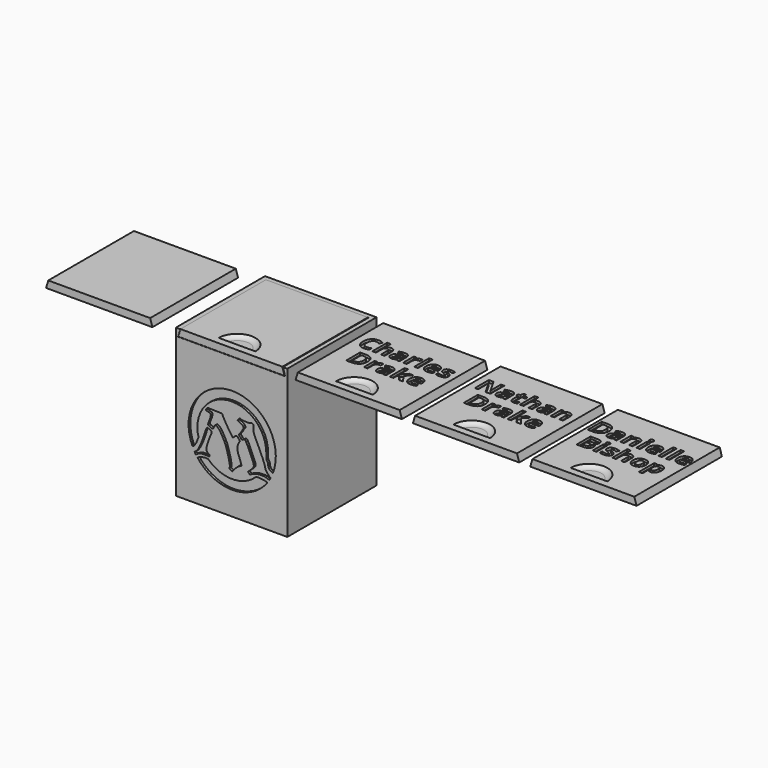
from build123d import *

# Parameters (mm, degrees)
F0_W          = 76
F0_H          = 76
F0_W_2        = 70
F0_H_2        = 70
F1_DEPTH      = 101
F2_T          = -3
F4_DEPTH      = 1.5
F6_DEPTH      = 1.5
F8_DEPTH      = 73
F10_DEPTH     = 73
F13_DEPTH     = 2
F14_T2_ANGLE  = 180
F15_DEPTH     = 0.2
F17_TEXT_SIZE = 16.6666666667
F18_DEPTH     = 1.7
F20_TEXT_SIZE = 16.6666666667
F21_DEPTH     = 1.7
F23_TEXT_SIZE = 16.6666666667
F24_DEPTH     = 1.7


# Not quite as in the source:
# - a fillet or chamfer that OpenCascade refuses, or shapes differently, is made with other operations: its cross-section is extruded or revolved along the edge and cut away or added
# - ends of sketch curves that miss each other by under 0.0002 mm in the source are joined
# - Text() gives the source's letters only with a copy of the font that has no kerning and outlines rounded to 1/6400 em; it was checked with that copy


with BuildPart() as f1:
    # F0 (on Top) → F1 (new body)
    with BuildSketch(Plane.XY):
        Rectangle(F0_W, F0_H)
        Rectangle(F0_W_2, F0_H_2, mode=Mode.SUBTRACT)
        Rectangle(F0_W_2, F0_H_2)
    extrude(amount=F1_DEPTH)

    # F2
    f2_openings = [f1.faces().sort_by_distance(p)[0] for p in [
        (0, 0, 101),
    ]]
    offset(amount=F2_T, openings=f2_openings)

    # F3 (on face) → F4 (cut)
    with BuildSketch(Plane.XZ.offset(38)):
        Polygon((-0.4040717683, 75.5102922818), (-4.3064167683, 75.1443172818), (-8.1267827683, 74.2684942818), (-11.7988487683, 72.8980352818), (-15.2588887683, 71.0567302818), (-18.4468317683, 68.7765432818), (-21.3073387683, 66.0970412818), (-23.7907747683, 63.0647482818), (-25.8540087683, 59.7322922818), (-27.4612537683, 56.1575202818), (-28.5845947683, 52.4024732818), (-29.2045377683, 48.5323482818), (-29.3103197683, 44.6143062818), (-28.9001077683, 40.7163642818), (-27.9810187683, 36.9061802818), (-26.6491757683, 33.4574742818), (-26.3627217683, 33.5535842818), (-26.1486297683, 33.6569762818), (-25.9661717683, 33.7809942818), (-25.2596027683, 34.5743172818), (-24.0698427683, 36.3678992818), (-22.4587547683, 40.3571682818), (-23.0023267683, 42.0458712818), (-23.3073607683, 43.9042412818), (-23.3334187683, 45.7713752818), (-23.3314467683, 46.0294862818), (-23.3266527683, 46.2869182818), (-23.3085647683, 46.8008852818), (-23.2385757683, 47.8249932818), (-23.0833227683, 49.1302592818), (-22.3553197683, 52.4062522818), (-21.1616097683, 55.5485932818), (-19.5282317683, 58.4865122818), (-17.4891687683, 61.1588742818), (-15.0868497683, 63.5100752818), (-12.3712617683, 65.4912032818), (-9.3989017683, 67.0610272818), (-6.2316137683, 68.1868982818), (-2.9439647683, 68.8436392818), (-2.8517567683, 68.8550622818), (-2.7680227683, 68.8651182818), (-2.6006807683, 68.8843102818), (-2.2602087683, 68.9196172818), (0.4207302317, 69.0225062818), (3.7255052317, 68.7861422818), (6.9670582317, 68.0809872818), (10.0752632317, 66.9216932818), (12.9868392317, 65.3318452818), (15.6425272317, 63.3438232818), (17.9882562317, 60.9980982818), (19.9762742317, 58.3424102818), (21.5661222317, 55.4308302818), (22.7254202317, 52.3226262818), (23.4287152317, 49.0896022818), (23.4416052317, 48.9988102818), (23.4530092317, 48.9163652818), (23.4749022317, 48.7515842818), (23.5158092317, 48.4162602818), (23.6666292317, 45.7787222818), (23.6513842317, 42.5201402818), (23.6885372317, 42.1498222818), (23.7861742317, 41.8070362818), (24.1682732317, 41.1271972818), (24.6231682317, 40.4245682818), (24.7742252317, 40.0015192818), (24.8532512317, 39.5750872818), (25.0745872317, 37.9653192818), (25.3304182317, 37.2385912818), (25.5115312317, 36.9209862818), (25.7367912317, 36.6349522818), (26.3194922317, 36.1164552818), (26.9907082317, 35.6731752818), (28.1405202317, 35.0311852818), (29.2599612317, 38.4858372818), (29.9675152317, 42.3409122818), (30.1621242317, 46.2555522818), (29.8404132317, 50.1617952818), (29.0079742317, 53.9918382818), (27.6792442317, 57.6792162818), (25.8772982317, 61.1599112818), (23.6334062317, 64.3734962818), (20.9865192317, 67.2642132818), (17.9825872317, 69.7818692818), (14.6737442317, 71.8827712818), (11.1174252317, 73.5304482818), (7.3753592317, 74.6963022818), (3.5125112317, 75.3600862818), align=None)
        Polygon((6.6751642317, 32.9071462818), (6.6608672317, 32.9569952818), (6.6454502317, 33.0107452818), (6.6146502317, 33.1180932818), (6.5538172317, 33.3295452818), (5.6720412317, 36.0862752818), (4.4881632317, 39.2291942818), (4.0456822317, 40.8744592818), (3.9273242317, 41.7380692818), (3.9263262317, 42.6140772818), (4.0560452317, 43.4793802818), (4.3012332317, 44.3147342818), (4.9789142317, 45.8947672818), (5.5673262317, 46.7298182818), (5.5872702317, 46.7855902818), (5.5946772317, 46.8564762818), (5.5749522317, 47.0902502818), (5.5417852317, 47.3312342818), (5.5148902317, 47.4229682818), (5.4906342317, 47.4574172818), (4.1636202317, 48.9975312818), (3.9991122317, 49.1464282818), (3.8212272317, 49.2624842818), (3.6371602317, 49.3319992818), (3.4438702317, 49.3514842818), (2.9793182317, 49.2897472818), (2.7750402317, 49.2257002818), (2.5926592317, 49.1334292818), (0.8799152317, 47.6042772818), (0.2146652317, 48.4917962818), (-1.6956667683, 51.1786762818), (-3.4535407683, 53.9708882818), (-5.1146707683, 56.8205992818), (-6.5391337683, 59.6266332818), (-16.4574717683, 59.9183512818), (-17.3783847683, 58.6290542818), (-17.6114987683, 58.2852152818), (-17.5473197683, 58.2122772818), (-17.2430877683, 57.9413892818), (-17.1002837683, 57.8581352818), (-16.9522457683, 57.8031692818), (-16.1054727683, 57.6989872818), (-15.2653657683, 57.4011922818), (-14.8346957683, 57.1973742818), (-14.6073227683, 57.0759572818), (-14.3969047683, 56.9171192818), (-14.2963787683, 56.7989642818), (-14.2235407683, 56.6640842818), (-14.1829787683, 56.5193962818), (-14.1671697683, 56.3697062818), (-14.2065517683, 55.8781422818), (-14.5779357683, 54.1757612818), (-15.2036547683, 52.5433812818), (-15.8162127683, 50.9462142818), (-15.9550077683, 50.5445352818), (-16.0361087683, 50.1631322818), (-16.0298377683, 50.0151142818), (-15.9856117683, 49.8680142818), (-15.9031267683, 49.7260382818), (-15.7900397683, 49.6017142818), (-15.6523917683, 49.5030882818), (-15.4873997683, 49.4226182818), (-15.0883547683, 49.2697922818), (-14.2998287683, 48.9139002818), (-13.5130627683, 48.5047732818), (-13.3405107683, 48.4386472818), (-13.1764937683, 48.4053592818), (-13.1134217683, 48.4038392818), (-13.0535567683, 48.4109422818), (-12.9014757683, 48.4612962818), (-12.7527247683, 48.5495352818), (-12.6178257683, 48.6648692818), (-12.3813457683, 48.9753872818), (-12.0048267683, 49.7100382818), (-11.6465307683, 50.5380912818), (-11.5449677683, 50.7636942818), (-11.4653817683, 50.8848622818), (-11.3646547683, 50.9928432818), (-11.2350897683, 51.0807082818), (-11.0845497683, 51.1331702818), (-10.9318587683, 51.1503912818), (-10.7798917683, 51.1432752818), (-10.5186387683, 51.0872102818), (-10.2778097683, 50.9907612818), (-9.8805267683, 50.7485262818), (-9.1811767683, 50.1877902818), (-7.9924437683, 48.8806012818), (-6.2182927683, 45.8939282818), (-4.9789597683, 43.5191462818), (-3.8746507683, 41.0665042818), (-2.3727067683, 35.9256042818), (-1.7384157683, 33.3403722818), (-1.2292867683, 30.6815502818), (-1.1727277683, 29.9759482818), (-1.2474887683, 29.2811342818), (-1.4100077683, 28.6041812818), (-1.4760157683, 28.4177382818), (-1.5646707683, 28.2511322818), (-1.5909377683, 28.2048122818), (-1.4712677683, 28.1729212818), (-1.1100707683, 28.0248972818), (-0.5449877683, 27.6707032818), (0.0221042317, 27.3344842818), (0.3247722317, 27.1199452818), (0.4369792317, 26.9996132818), (0.5893612317, 27.3901922818), (0.8999862317, 27.8839222818), (1.6747112317, 28.6821742818), (3.1945492317, 30.2222592818), (3.9915072317, 30.9908082818), (4.9131732317, 31.5827902818), (5.8692902317, 32.1576632818), (6.1356392317, 32.2904342818), (6.4263152317, 32.3874972818), (6.7308582317, 32.4260882818), (6.7661262317, 32.4256062818), (6.7659022317, 32.5469872818), align=None)
        Polygon((19.4331262317, 45.6693772818), (18.7905172317, 47.0654182818), (16.2318482317, 52.3506892818), (15.1644112317, 55.0983982818), (14.9473782317, 55.8312792818), (14.8689412317, 56.6017252818), (14.9362672317, 58.0945852818), (15.0656712317, 59.5406802818), (15.0657572317, 59.7102412818), (15.0465212317, 59.8561612818), (15.0290602317, 59.9060242818), (14.9943362317, 59.9406242818), (14.9481502317, 59.9726752818), (14.3079202317, 60.3253332818), (14.0012052317, 60.5074992818), (13.9527942317, 60.5289102818), (13.9119982317, 60.5386352818), (13.8657752317, 60.5407872818), (13.8229512317, 60.5363292818), (13.1155542317, 60.2902882818), (11.6562662317, 60.0146172818), (10.1606882317, 59.9238292818), (8.6832032317, 60.0608922818), (7.1986622317, 60.1859402818), (5.7808482317, 60.6009662818), (5.6320202317, 60.6314572818), (5.5014052317, 60.6331252818), (5.4675822317, 60.6252572818), (5.4331542317, 60.6097732818), (5.3273292317, 60.5312812818), (4.8500532317, 59.9977642818), (4.3934102317, 59.4557892818), (4.2193062317, 59.1814072818), (4.1707162317, 59.0522822818), (4.1465932317, 58.9122982818), (4.1488822317, 58.8632422818), (4.1756692317, 58.8402332818), (4.3037862317, 58.7754472818), (4.4883272317, 58.7116562818), (5.2434032317, 58.4221502818), (6.5230432317, 57.7417082818), (7.1513012317, 57.3604402818), (7.4752972317, 57.1388062818), (7.7765062317, 56.8636292818), (8.0220052317, 56.5262402818), (8.1952242317, 56.1418132818), (8.2518352317, 55.9184262818), (8.2693342317, 55.6885632818), (8.2346242317, 55.4615802818), (8.1506472317, 55.2412382818), (7.2537562317, 54.0066212818), (6.5438492317, 52.7462712818), (6.1004322317, 52.1138612818), (5.5254822317, 51.5674102818), (5.2518382317, 51.3216692818), (5.1587992317, 51.2121672818), (5.0934362317, 51.1030722818), (5.0563012317, 50.9904402818), (5.0456822317, 50.8624742818), (5.0619862317, 50.7251232818), (5.1023522317, 50.5949512818), (5.2591022317, 50.3069972818), (5.4589892317, 50.0274912818), (5.9121182317, 49.4785182818), (6.4025522317, 48.9393162818), (6.6525292317, 48.6829932818), (6.7698002317, 48.5869832818), (6.8877992317, 48.5156942818), (7.0169432317, 48.4675752818), (7.1683632317, 48.4341952818), (7.5121262317, 48.3911902818), (7.5647132317, 48.3935052818), (7.6128132317, 48.4023992818), (7.6542592317, 48.4180422818), (7.6940762317, 48.4412912818), (7.9739342317, 48.6789562818), (8.3147012317, 48.9021112818), (8.5317432317, 48.9879102818), (8.6601542317, 49.0161072818), (8.7927192317, 49.0248262818), (8.9276212317, 49.0086632818), (9.0615762317, 48.9674112818), (9.2705782317, 48.8508882818), (9.4471912317, 48.6982772818), (9.5963252317, 48.5211472818), (10.9501062317, 45.8788312818), (14.8118052317, 36.9356832818), (15.1745822317, 35.7297962818), (15.2007112317, 35.3804292818), (15.1718342317, 35.0381422818), (15.0947432317, 34.7059992818), (14.9739262317, 34.3865492818), (14.6478182317, 33.8273462818), (14.2412732317, 33.3228582818), (13.3561822317, 32.4385592818), (11.5900882317, 30.8298382818), (11.3804882317, 30.6068212818), (11.2804402317, 30.4923272818), (11.2343352317, 30.4290342818), (11.4540852317, 30.2101272818), (11.9326672317, 29.7310812818), (12.2636792317, 29.2794712818), (12.5302522317, 29.0761602818), (13.6507782317, 29.7814472818), (15.0438642317, 30.3694292818), (16.4672942317, 30.8459912818), (17.9437402317, 31.1700302818), (19.9820472317, 31.3222472818), (22.0387242317, 31.3013952818), (24.0452282317, 30.8220302818), (25.7646972317, 30.2022802818), (26.0578182317, 30.6861072818), (26.4382662317, 31.3522482818), (26.6824652317, 31.8066462818), (26.1440332317, 32.0837282818), (25.4514272317, 32.6360592818), (24.3573592317, 33.9509892818), (23.3797372317, 35.3647242818), (23.0557862317, 36.1783372818), (22.8748422317, 37.0074102818), (22.2124702317, 39.0857212818), (21.2855852317, 41.4764132818), align=None)
        Polygon((24.4773142317, 28.3088662818), (23.8207522317, 28.5389362818), (22.8023862317, 28.7482302818), (20.6941912317, 29.0297302818), (18.5800212317, 29.3093132818), (17.5534582317, 29.2993892818), (16.6022162317, 29.0879432818), (14.1644562317, 27.0214872818), (11.3933272317, 25.2757592818), (8.4043872317, 23.9367142818), (5.2569512317, 23.0309612818), (2.0134682317, 22.5764432818), (-1.2616947683, 22.5821942818), (-4.5035707683, 23.0480862818), (-7.6478027683, 23.9648982818), (-10.6320197683, 25.3144162818), (-13.3970037683, 27.0698672818), (-15.8302047683, 29.1471782818), (-16.7546557683, 29.3824352818), (-17.7254377683, 29.4338512818), (-19.7580277683, 29.1214912818), (-21.7231527683, 28.5883942818), (-22.5988087683, 28.1437902818), (-23.2128767683, 27.7230022818), (-20.9627687683, 25.0850702818), (-18.2065577683, 22.5727732818), (-15.1576687683, 20.4250672818), (-11.8640407683, 18.6756872818), (-8.3774187683, 17.3521212818), (-4.7525907683, 16.4751892818), (-1.0465357683, 16.0586582818), (2.6825072317, 16.1090752818), (6.3759462317, 16.6256492818), (9.9757372317, 17.6002622818), (13.4253012317, 19.0175982818), (16.6704352317, 20.8553832818), (19.6601432317, 23.0847432818), (22.3474262317, 25.6706302818), align=None)
        Polygon((-25.0980437683, 30.8046492818), (-25.2241227683, 30.7627782818), (-25.2725437683, 30.7408502818), (-24.8979357683, 29.7951742818), (-24.4477487683, 29.1557772818), (-24.1651227683, 29.4026772818), (-23.7359097683, 29.6720222818), (-22.8871427683, 30.1942022818), (-21.0300087683, 30.8732472818), (-20.0450237683, 31.0837882818), (-19.0547127683, 31.1374072818), (-17.0978867683, 31.1274692818), (-14.9320787683, 30.9441102818), (-14.9283877683, 31.6998682818), (-14.9593187683, 31.9267422818), (-14.9844177683, 32.0097652818), (-15.0212367683, 32.0800272818), (-15.0751587683, 32.1458972818), (-15.1449537683, 32.2080712818), (-15.3449557683, 32.3361442818), (-16.2849107683, 32.8504562818), (-16.6852527683, 33.2939272818), (-16.9767747683, 33.8013592818), (-17.1642547683, 34.3475072818), (-17.2369137683, 34.9231002818), (-17.0860877683, 36.0103432818), (-16.4812087683, 38.0341712818), (-15.1390857683, 42.0066832818), (-13.5565947683, 45.8275382818), (-13.5383627683, 46.2129562818), (-13.5691997683, 46.3795032818), (-13.5909727683, 46.4294732818), (-13.6209857683, 46.4718842818), (-13.7531897683, 46.5867042818), (-13.9315137683, 46.7011812818), (-14.3148647683, 46.9373762818), (-14.4489887683, 47.0177382818), (-14.5819327683, 47.0952882818), (-14.8495357683, 47.2429052818), (-15.4132607683, 47.5133822818), (-15.8733647683, 47.7120992818), (-16.2711577683, 47.8688382818), (-16.3399887683, 47.8798172818), (-16.4219987683, 47.8816622818), (-16.5053437683, 47.8724262818), (-16.5866377683, 47.8524302818), (-16.6620077683, 47.8226722818), (-16.7225117683, 47.7879752818), (-16.8481937683, 47.6751812818), (-17.0781837683, 47.3335572818), (-17.7951467683, 45.6839642818), (-19.1565487683, 41.4368052818), (-20.7460367683, 37.2350202818), (-21.5742747683, 35.3318482818), (-22.5395037683, 33.4935902818), (-23.7372817683, 31.7584062818), (-24.5687447683, 31.0810082818), (-24.8143747683, 30.9182372818), align=None)
    extrude(amount=-F4_DEPTH, mode=Mode.SUBTRACT)

    # F5 (on face) → F6 (cut)
    with BuildSketch(Plane(origin=(0, 38, 0), x_dir=(-1, 0, 0), z_dir=(0, 1, 0))):
        Polygon((0.0653751924, 80.0444194725), (-3.8369698076, 79.6784444725), (-7.6573358076, 78.8026214725), (-11.3294018076, 77.4321624725), (-14.7894418076, 75.5908574725), (-17.9773848076, 73.3106704725), (-20.8378918076, 70.6311684725), (-23.3213278076, 67.5988754725), (-25.3845618076, 64.2664194725), (-26.9918068076, 60.6916474725), (-28.1151478076, 56.9366004725), (-28.7350908076, 53.0664754725), (-28.8408728076, 49.1484334725), (-28.4306608076, 45.2504914725), (-27.5115718076, 41.4403074725), (-26.1797288076, 37.9916014725), (-25.8932748076, 38.0877114725), (-25.6791828076, 38.1911034725), (-25.4967248076, 38.3151214725), (-24.7901558076, 39.1084444725), (-23.6003958076, 40.9020264725), (-21.9893078076, 44.8912954725), (-22.5328798076, 46.5799984725), (-22.8379138076, 48.4383684725), (-22.8639718076, 50.3055024725), (-22.8619998076, 50.5636134725), (-22.8572058076, 50.8210454725), (-22.8391178076, 51.3350124725), (-22.7691288076, 52.3591204725), (-22.6138758076, 53.6643864725), (-21.8858728076, 56.9403794725), (-20.6921628076, 60.0827204725), (-19.0587848076, 63.0206394725), (-17.0197218076, 65.6930014725), (-14.6174028076, 68.0442024725), (-11.9018148076, 70.0253304725), (-8.9294548076, 71.5951544725), (-5.7621668076, 72.7210254725), (-2.4745178076, 73.3777664725), (-2.3823098076, 73.3891894725), (-2.2985758076, 73.3992454725), (-2.1312338076, 73.4184374725), (-1.7907618076, 73.4537444725), (0.8901771924, 73.5566334725), (4.1949521924, 73.3202694725), (7.4365051924, 72.6151144725), (10.5447101924, 71.4558204725), (13.4562861924, 69.8659724725), (16.1119741924, 67.8779504725), (18.4577031924, 65.5322254725), (20.4457211924, 62.8765374725), (22.0355691924, 59.9649574725), (23.1948671924, 56.8567534725), (23.8981621924, 53.6237294725), (23.9110521924, 53.5329374725), (23.9224561924, 53.4504924725), (23.9443491924, 53.2857114725), (23.9852561924, 52.9503874725), (24.1360761924, 50.3128494725), (24.1208311924, 47.0542674725), (24.1579841924, 46.6839494725), (24.2556211924, 46.3411634725), (24.6377201924, 45.6613244725), (25.0926151924, 44.9586954725), (25.2436721924, 44.5356464725), (25.3226981924, 44.1092144725), (25.5440341924, 42.4994464725), (25.7998651924, 41.7727184725), (25.9809781924, 41.4551134725), (26.2062381924, 41.1690794725), (26.7889391924, 40.6505824725), (27.4601551924, 40.2073024725), (28.6099671924, 39.5653124725), (29.7294081924, 43.0199644725), (30.4369621924, 46.8750394725), (30.6315711924, 50.7896794725), (30.3098601924, 54.6959224725), (29.4774211924, 58.5259654725), (28.1486911924, 62.2133434725), (26.3467451924, 65.6940384725), (24.1028531924, 68.9076234725), (21.4559661924, 71.7983404725), (18.4520341924, 74.3159964725), (15.1431911924, 76.4168984725), (11.5868721924, 78.0645754725), (7.8448061924, 79.2304294725), (3.9819581924, 79.8942134725), align=None)
        Polygon((7.1446111924, 37.4412734725), (7.1303141924, 37.4911224725), (7.1148971924, 37.5448724725), (7.0840971924, 37.6522204725), (7.0232641924, 37.8636724725), (6.1414881924, 40.6204024725), (4.9576101924, 43.7633214725), (4.5151291924, 45.4085864725), (4.3967711924, 46.2721964725), (4.3957731924, 47.1482044725), (4.5254921924, 48.0135074725), (4.7706801924, 48.8488614725), (5.4483611924, 50.4288944725), (6.0367731924, 51.2639454725), (6.0567171924, 51.3197174725), (6.0641241924, 51.3906034725), (6.0443991924, 51.6243774725), (6.0112321924, 51.8653614725), (5.9843371924, 51.9570954725), (5.9600811924, 51.9915444725), (4.6330671924, 53.5316584725), (4.4685591924, 53.6805554725), (4.2906741924, 53.7966114725), (4.1066071924, 53.8661264725), (3.9133171924, 53.8856114725), (3.4487651924, 53.8238744725), (3.2444871924, 53.7598274725), (3.0621061924, 53.6675564725), (1.3493621924, 52.1384044725), (0.6841121924, 53.0259234725), (-1.2262198076, 55.7128034725), (-2.9840938076, 58.5050154725), (-4.6452238076, 61.3547264725), (-6.0696868076, 64.1607604725), (-15.9880248076, 64.4524784725), (-16.9089378076, 63.1631814725), (-17.1420518076, 62.8193424725), (-17.0778728076, 62.7464044725), (-16.7736408076, 62.4755164725), (-16.6308368076, 62.3922624725), (-16.4827988076, 62.3372964725), (-15.6360258076, 62.2331144725), (-14.7959188076, 61.9353194725), (-14.3652488076, 61.7315014725), (-14.1378758076, 61.6100844725), (-13.9274578076, 61.4512464725), (-13.8269318076, 61.3330914725), (-13.7540938076, 61.1982114725), (-13.7135318076, 61.0535234725), (-13.6977228076, 60.9038334725), (-13.7371048076, 60.4122694725), (-14.1084888076, 58.7098884725), (-14.7342078076, 57.0775084725), (-15.3467658076, 55.4803414725), (-15.4855608076, 55.0786624725), (-15.5666618076, 54.6972594725), (-15.5603908076, 54.5492414725), (-15.5161648076, 54.4021414725), (-15.4336798076, 54.2601654725), (-15.3205928076, 54.1358414725), (-15.1829448076, 54.0372154725), (-15.0179528076, 53.9567454725), (-14.6189078076, 53.8039194725), (-13.8303818076, 53.4480274725), (-13.0436158076, 53.0389004725), (-12.8710638076, 52.9727744725), (-12.7070468076, 52.9394864725), (-12.6439748076, 52.9379664725), (-12.5841098076, 52.9450694725), (-12.4320288076, 52.9954234725), (-12.2832778076, 53.0836624725), (-12.1483788076, 53.1989964725), (-11.9118988076, 53.5095144725), (-11.5353798076, 54.2441654725), (-11.1770838076, 55.0722184725), (-11.0755208076, 55.2978214725), (-10.9959348076, 55.4189894725), (-10.8952078076, 55.5269704725), (-10.7656428076, 55.6148354725), (-10.6151028076, 55.6672974725), (-10.4624118076, 55.6845184725), (-10.3104448076, 55.6774024725), (-10.0491918076, 55.6213374725), (-9.8083628076, 55.5248884725), (-9.4110798076, 55.2826534725), (-8.7117298076, 54.7219174725), (-7.5229968076, 53.4147284725), (-5.7488458076, 50.4280554725), (-4.5095128076, 48.0532734725), (-3.4052038076, 45.6006314725), (-1.9032598076, 40.4597314725), (-1.2689688076, 37.8744994725), (-0.7598398076, 35.2156774725), (-0.7032808076, 34.5100754725), (-0.7780418076, 33.8152614725), (-0.9405608076, 33.1383084725), (-1.0065688076, 32.9518654725), (-1.0952238076, 32.7852594725), (-1.1214908076, 32.7389394725), (-1.0018208076, 32.7070484725), (-0.6406238076, 32.5590244725), (-0.0755408076, 32.2048304725), (0.4915511924, 31.8686114725), (0.7942191924, 31.6540724725), (0.9064261924, 31.5337404725), (1.0588081924, 31.9243194725), (1.3694331924, 32.4180494725), (2.1441581924, 33.2163014725), (3.6639961924, 34.7563864725), (4.4609541924, 35.5249354725), (5.3826201924, 36.1169174725), (6.3387371924, 36.6917904725), (6.6050861924, 36.8245614725), (6.8957621924, 36.9216244725), (7.2003051924, 36.9602154725), (7.2355731924, 36.9597334725), (7.2353491924, 37.0811144725), align=None)
        Polygon((19.9025731924, 50.2035044725), (19.2599641924, 51.5995454725), (16.7012951924, 56.8848164725), (15.6338581924, 59.6325254725), (15.4168251924, 60.3654064725), (15.3383881924, 61.1358524725), (15.4057141924, 62.6287124725), (15.5351181924, 64.0748074725), (15.5352041924, 64.2443684725), (15.5159681924, 64.3902884725), (15.4985071924, 64.4401514725), (15.4637831924, 64.4747514725), (15.4175971924, 64.5068024725), (14.7773671924, 64.8594604725), (14.4706521924, 65.0416264725), (14.4222411924, 65.0630374725), (14.3814451924, 65.0727624725), (14.3352221924, 65.0749144725), (14.2923981924, 65.0704564725), (13.5850011924, 64.8244154725), (12.1257131924, 64.5487444725), (10.6301351924, 64.4579564725), (9.1526501924, 64.5950194725), (7.6681091924, 64.7200674725), (6.2502951924, 65.1350934725), (6.1014671924, 65.1655844725), (5.9708521924, 65.1672524725), (5.9370291924, 65.1593844725), (5.9026011924, 65.1439004725), (5.7967761924, 65.0654084725), (5.3195001924, 64.5318914725), (4.8628571924, 63.9899164725), (4.6887531924, 63.7155344725), (4.6401631924, 63.5864094725), (4.6160401924, 63.4464254725), (4.6183291924, 63.3973694725), (4.6451161924, 63.3743604725), (4.7732331924, 63.3095744725), (4.9577741924, 63.2457834725), (5.7128501924, 62.9562774725), (6.9924901924, 62.2758354725), (7.6207481924, 61.8945674725), (7.9447441924, 61.6729334725), (8.2459531924, 61.3977564725), (8.4914521924, 61.0603674725), (8.6646711924, 60.6759404725), (8.7212821924, 60.4525534725), (8.7387811924, 60.2226904725), (8.7040711924, 59.9957074725), (8.6200941924, 59.7753654725), (7.7232031924, 58.5407484725), (7.0132961924, 57.2803984725), (6.5698791924, 56.6479884725), (5.9949291924, 56.1015374725), (5.7212851924, 55.8557964725), (5.6282461924, 55.7462944725), (5.5628831924, 55.6371994725), (5.5257481924, 55.5245674725), (5.5151291924, 55.3966014725), (5.5314331924, 55.2592504725), (5.5717991924, 55.1290784725), (5.7285491924, 54.8411244725), (5.9284361924, 54.5616184725), (6.3815651924, 54.0126454725), (6.8719991924, 53.4734434725), (7.1219761924, 53.2171204725), (7.2392471924, 53.1211104725), (7.3572461924, 53.0498214725), (7.4863901924, 53.0017024725), (7.6378101924, 52.9683224725), (7.9815731924, 52.9253174725), (8.0341601924, 52.9276324725), (8.0822601924, 52.9365264725), (8.1237061924, 52.9521694725), (8.1635231924, 52.9754184725), (8.4433811924, 53.2130834725), (8.7841481924, 53.4362384725), (9.0011901924, 53.5220374725), (9.1296011924, 53.5502344725), (9.2621661924, 53.5589534725), (9.3970681924, 53.5427904725), (9.5310231924, 53.5015384725), (9.7400251924, 53.3850154725), (9.9166381924, 53.2324044725), (10.0657721924, 53.0552744725), (11.4195531924, 50.4129584725), (15.2812521924, 41.4698104725), (15.6440291924, 40.2639234725), (15.6701581924, 39.9145564725), (15.6412811924, 39.5722694725), (15.5641901924, 39.2401264725), (15.4433731924, 38.9206764725), (15.1172651924, 38.3614734725), (14.7107201924, 37.8569854725), (13.8256291924, 36.9726864725), (12.0595351924, 35.3639654725), (11.8499351924, 35.1409484725), (11.7498871924, 35.0264544725), (11.7037821924, 34.9631614725), (11.9235321924, 34.7442544725), (12.4021141924, 34.2652084725), (12.7331261924, 33.8135984725), (12.9996991924, 33.6102874725), (14.1202251924, 34.3155744725), (15.5133111924, 34.9035564725), (16.9367411924, 35.3801184725), (18.4131871924, 35.7041574725), (20.4514941924, 35.8563744725), (22.5081711924, 35.8355224725), (24.5146751924, 35.3561574725), (26.2341441924, 34.7364074725), (26.5272651924, 35.2202344725), (26.9077131924, 35.8863754725), (27.1519121924, 36.3407734725), (26.6134801924, 36.6178554725), (25.9208741924, 37.1701864725), (24.8268061924, 38.4851164725), (23.8491841924, 39.8988514725), (23.5252331924, 40.7124644725), (23.3442891924, 41.5415374725), (22.6819171924, 43.6198484725), (21.7550321924, 46.0105404725), align=None)
        Polygon((24.9467611924, 32.8429934725), (24.2901991924, 33.0730634725), (23.2718331924, 33.2823574725), (21.1636381924, 33.5638574725), (19.0494681924, 33.8434404725), (18.0229051924, 33.8335164725), (17.0716631924, 33.6220704725), (14.6339031924, 31.5556144725), (11.8627741924, 29.8098864725), (8.8738341924, 28.4708414725), (5.7263981924, 27.5650884725), (2.4829151924, 27.1105704725), (-0.7922478076, 27.1163214725), (-4.0341238076, 27.5822134725), (-7.1783558076, 28.4990254725), (-10.1625728076, 29.8485434725), (-12.9275568076, 31.6039944725), (-15.3607578076, 33.6813054725), (-16.2852088076, 33.9165624725), (-17.2559908076, 33.9679784725), (-19.2885808076, 33.6556184725), (-21.2537058076, 33.1225214725), (-22.1293618076, 32.6779174725), (-22.7434298076, 32.2571294725), (-20.4933218076, 29.6191974725), (-17.7371108076, 27.1069004725), (-14.6882218076, 24.9591944725), (-11.3945938076, 23.2098144725), (-7.9079718076, 21.8862484725), (-4.2831438076, 21.0093164725), (-0.5770888076, 20.5927854725), (3.1519541924, 20.6432024725), (6.8453931924, 21.1597764725), (10.4451841924, 22.1343894725), (13.8947481924, 23.5517254725), (17.1398821924, 25.3895104725), (20.1295901924, 27.6188704725), (22.8168731924, 30.2047574725), align=None)
        Polygon((-24.6285968076, 35.3387764725), (-24.7546758076, 35.2969054725), (-24.8030968076, 35.2749774725), (-24.4284888076, 34.3293014725), (-23.9783018076, 33.6899044725), (-23.6956758076, 33.9368044725), (-23.2664628076, 34.2061494725), (-22.4176958076, 34.7283294725), (-20.5605618076, 35.4073744725), (-19.5755768076, 35.6179154725), (-18.5852658076, 35.6715344725), (-16.6284398076, 35.6615964725), (-14.4626318076, 35.4782374725), (-14.4589408076, 36.2339954725), (-14.4898718076, 36.4608694725), (-14.5149708076, 36.5438924725), (-14.5517898076, 36.6141544725), (-14.6057118076, 36.6800244725), (-14.6755068076, 36.7421984725), (-14.8755088076, 36.8702714725), (-15.8154638076, 37.3845834725), (-16.2158058076, 37.8280544725), (-16.5073278076, 38.3354864725), (-16.6948078076, 38.8816344725), (-16.7674668076, 39.4572274725), (-16.6166408076, 40.5444704725), (-16.0117618076, 42.5682984725), (-14.6696388076, 46.5408104725), (-13.0871478076, 50.3616654725), (-13.0689158076, 50.7470834725), (-13.0997528076, 50.9136304725), (-13.1215258076, 50.9636004725), (-13.1515388076, 51.0060114725), (-13.2837428076, 51.1208314725), (-13.4620668076, 51.2353084725), (-13.8454178076, 51.4715034725), (-13.9795418076, 51.5518654725), (-14.1124858076, 51.6294154725), (-14.3800888076, 51.7770324725), (-14.9438138076, 52.0475094725), (-15.4039178076, 52.2462264725), (-15.8017108076, 52.4029654725), (-15.8705418076, 52.4139444725), (-15.9525518076, 52.4157894725), (-16.0358968076, 52.4065534725), (-16.1171908076, 52.3865574725), (-16.1925608076, 52.3567994725), (-16.2530648076, 52.3221024725), (-16.3787468076, 52.2093084725), (-16.6087368076, 51.8676844725), (-17.3256998076, 50.2180914725), (-18.6871018076, 45.9709324725), (-20.2765898076, 41.7691474725), (-21.1048278076, 39.8659754725), (-22.0700568076, 38.0277174725), (-23.2678348076, 36.2925334725), (-24.0992978076, 35.6151354725), (-24.3449278076, 35.4523644725), align=None)
    extrude(amount=-F6_DEPTH, mode=Mode.SUBTRACT)

    # F7 (on face) → F8 (cut, through all)
    with BuildSketch(Plane.XZ.offset(38)):
        Polygon((35, 101), (-35, 101), (-36.5, 96), (36.5, 96), align=None)
    extrude(amount=-F8_DEPTH, mode=Mode.SUBTRACT)


with BuildPart() as f10:
    # F9 (on face) → F10 (new body, through all)
    with BuildSketch(Plane.XZ.offset(38)):
        Polygon((34.4779846746, 101), (-35, 101), (-36.5, 96), (35.9779846746, 96), align=None)
    extrude(amount=-F10_DEPTH)


with BuildPart() as f11_1:
    # F11: copy of F10
    add(f10.part.moved(Location((-90, 0, 0))))


with BuildPart() as f10_1:
    add(f10.part)

    # F12 (on face) → F13 (cut)
    with BuildSketch(Plane.XY.offset(101)):
        with BuildLine():
            Line((-12.7610076625, -33), (12.2389923375, -33))
            ThreePointArc((12.2389923375, -33), (-0.2610076625, -20.5), (-12.7610076625, -33))
        make_face()
    extrude(amount=-F13_DEPTH, mode=Mode.SUBTRACT)

    # F14: fillet of radius 5 on 1 edges, made by hand

    # F14_s1 → F14_t2 (revolve)
    with BuildSketch(Plane.XZ.offset(33)):
        with BuildLine():
            ThreePointArc((12.2389923375, 101), (10.475060315, 99.527864045), (8.2389923375, 99))
            Line((8.2389923375, 99), (12.2389923375, 99))
            Line((12.2389923375, 99), (12.2389923375, 101))
        make_face()
    revolve(axis=Axis((-0.2610076625, -33, 99), (0, 0, 1)), revolution_arc=F14_T2_ANGLE)

    # F15 (cut): a face of the model
    f15_faces = [f10_1.faces().sort_by_distance(p)[0] for p in [
        (-0.2610076627, -38, 98.4823889054),
    ]]
    extrude(f15_faces, amount=-F15_DEPTH, mode=Mode.SUBTRACT)


with BuildPart() as f16_1:
    # F16: copy of F10
    add(f10_1.part.moved(Location((80, 0, 0))))

    # F17 (on face) → F18 (cut)
    with BuildSketch(Plane.XY.offset(101)):
        with Locations((48.8431590039, 6)):
            Text('Charles', F17_TEXT_SIZE, font='Open Sans', font_style=FontStyle.BOLD, text_align=(TextAlign.LEFT, TextAlign.BOTTOM))
        with Locations((55.0189402539, -11)):
            Text('Drake', F17_TEXT_SIZE, font='Open Sans', font_style=FontStyle.BOLD, text_align=(TextAlign.LEFT, TextAlign.BOTTOM))
    extrude(amount=-F18_DEPTH, mode=Mode.SUBTRACT)


with BuildPart() as f19_1:
    # F19: copy of F10
    add(f10_1.part.moved(Location((160, 0, 0))))

    # F20 (on face) → F21 (cut)
    with BuildSketch(Plane.XY.offset(101)):
        with Locations((128.4121694206, 7)):
            Text('Nathan', F20_TEXT_SIZE, font='Open Sans', font_style=FontStyle.BOLD, text_align=(TextAlign.LEFT, TextAlign.BOTTOM))
        with Locations((134.4785756706, -10)):
            Text('Drake', F20_TEXT_SIZE, font='Open Sans', font_style=FontStyle.BOLD, text_align=(TextAlign.LEFT, TextAlign.BOTTOM))
    extrude(amount=-F21_DEPTH, mode=Mode.SUBTRACT)


with BuildPart() as f22_1:
    # F22: copy of F10
    add(f10_1.part.moved(Location((240, 0, 0))))

    # F23 (on face) → F24 (cut)
    with BuildSketch(Plane.XY.offset(101)):
        with Locations((205.4017527539, 7)):
            Text('Danielle', F23_TEXT_SIZE, font='Open Sans', font_style=FontStyle.BOLD, text_align=(TextAlign.LEFT, TextAlign.BOTTOM))
        with Locations((211.3783152539, -10)):
            Text('Bishop', F23_TEXT_SIZE, font='Open Sans', font_style=FontStyle.BOLD, text_align=(TextAlign.LEFT, TextAlign.BOTTOM))
    extrude(amount=-F24_DEPTH, mode=Mode.SUBTRACT)


solid = Compound([f1.part, f11_1.part, f10_1.part, f16_1.part, f19_1.part, f22_1.part])
